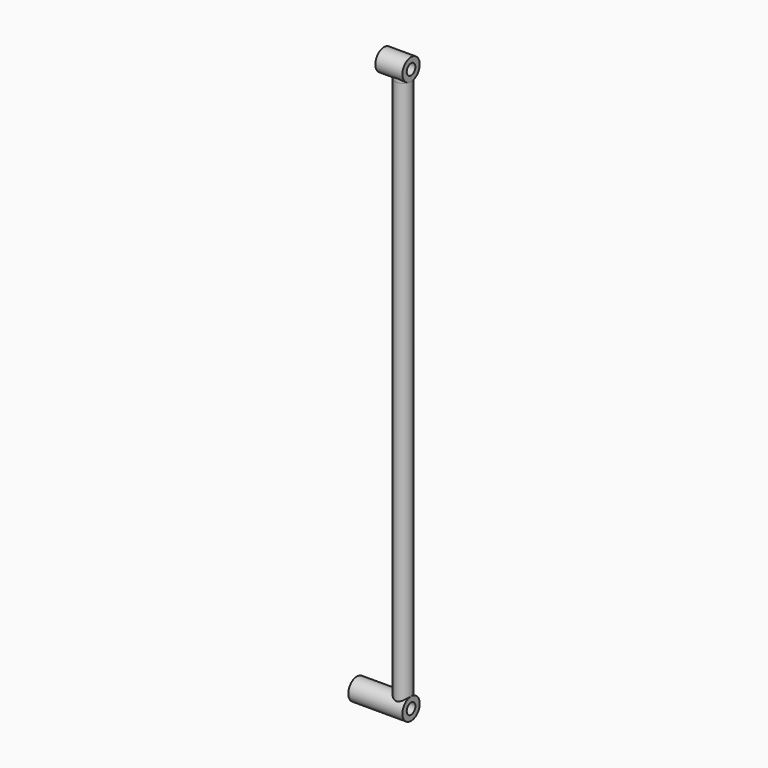
from build123d import *

# Parameters (mm, degrees)
F0_R          = 1.5
F1_DEPTH      = 100
F1_DEPTH_BACK = 0.75
F2_W          = 10
F2_H          = 1
F2_W_2        = 5
F5_DEPTH      = 1


with BuildPart() as f1:
    # F0 (on Top) → F1 (new body, two sides)
    with BuildSketch(Plane.XY) as f1_sk:
        Circle(F0_R)
    extrude(amount=F1_DEPTH)
    extrude(f1_sk.sketch, amount=-F1_DEPTH_BACK)

    # F2 (on Front) → F3 (revolve)
    with BuildSketch(Plane.XZ):
        with Locations((-3.5, -0.5)):
            Rectangle(F2_W, F2_H)
    revolve(axis=Axis((1.1637299322, 0, -2), (1, 0, 0)))

    # F5 (add): a face of the model
    f5_faces = [f1.faces().sort_by_distance(p)[0] for p in [
        (0, 0, 100),
    ]]


with BuildPart() as f4:
    # F2 (on Front) → F4 (revolve)
    with BuildSketch(Plane.XZ):
        with Locations((-1, 100.5)):
            Rectangle(F2_W_2, F2_H)
    revolve(axis=Axis((1.1637299322, 0, 102), (1, 0, 0)))


with BuildPart() as f1_1:
    add(f1.part)

    add(f4.part)  # F5 merges F4
    extrude(f5_faces, amount=F5_DEPTH)


solid = f1_1.part
